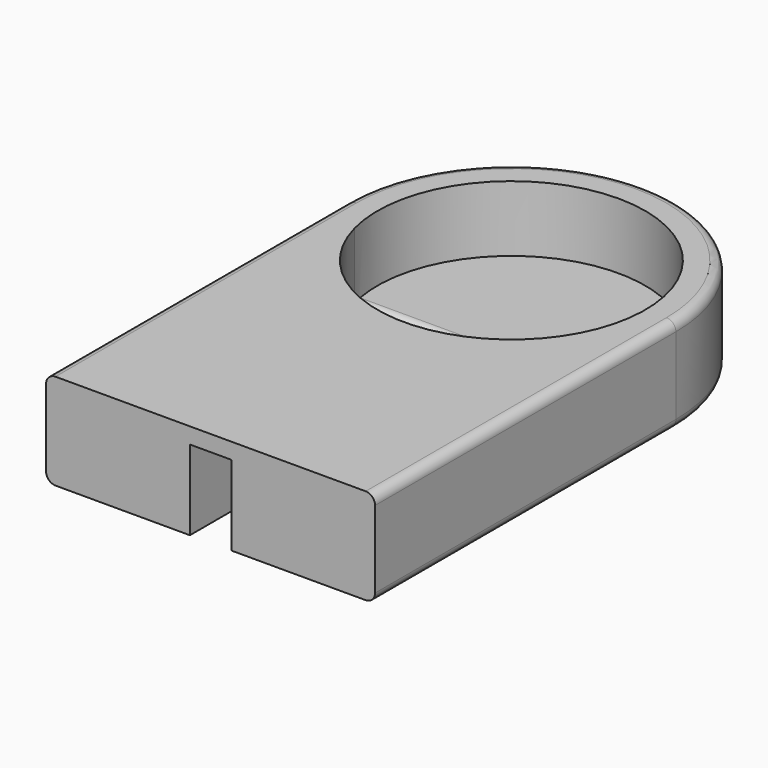
from build123d import *

# Parameters (mm, degrees)
F1_DEPTH     = 10.2
F2_R         = 14.25
F3_DEPTH     = 7
F4_W         = 4.4
F4_H         = 30
F5_DEPTH     = 8.5
F7_DEPTH     = 25
F9_T1_DEPTH  = 42.5
F9_T4_ANGLE  = 180
F9_T6_ANGLE  = 180
F9_T10_DEPTH = 32.5676095837
F9_S11_R     = 14.25
F9_T12_DEPTH = 18


# Not quite as in the source:
# - a fillet or chamfer that OpenCascade refuses, or shapes differently, is made with other operations: its cross-section is extruded or revolved along the edge and cut away or added


with BuildPart() as f1:
    # F0 (on Top) → F1 (new body)
    with BuildSketch(Plane.XY):
        with BuildLine():
            Line((-17.5, 20), (-17.5, -20))
            Line((-17.5, -20), (17.5, -20))
            Line((17.5, -20), (17.5, 20))
            ThreePointArc((17.5, 20), (0, 2.5), (-17.5, 20))
        make_face()
        with BuildLine():
            Line((17.5, 20), (-17.5, 20))
            ThreePointArc((-17.5, 20), (0, 2.5), (17.5, 20))
        make_face()
        with BuildLine():
            ThreePointArc((17.5, 20), (0, 37.5), (-17.5, 20))
            Line((-17.5, 20), (17.5, 20))
        make_face()
    extrude(amount=-F1_DEPTH)


with BuildPart() as f3:
    # F2 (on Top) → F3 (new body)
    with BuildSketch(Plane.XY):
        with Locations((0, 20)):
            Circle(F2_R)
    extrude(amount=-F3_DEPTH)


with BuildPart() as f5:
    # F4 (on face) → F5 (new body)
    with BuildSketch(Plane(origin=(0, 0, -10.2), x_dir=(1, 0, 0), z_dir=(0, 0, -1))):
        with Locations((0, 5)):
            Rectangle(F4_W, F4_H)
    extrude(amount=-F5_DEPTH)


with BuildPart() as f7:
    # F6 (on face) → F7 (new body)
    with BuildSketch(Plane(origin=(0, 0, -10.2), x_dir=(1, 0, 0), z_dir=(0, 0, -1))):
        with BuildLine():
            Line((-13.7838047919, -16.3848616264), (13.7838047919, -16.3848616264))
            ThreePointArc((13.7838047919, -16.3848616264), (0, -5.75), (-13.7838047919, -16.3848616264))
        make_face()
    extrude(amount=-F7_DEPTH)


with BuildPart() as f1_1:
    add(f1.part)

    # F8: cut F7, F5, F3
    add(f7.part, mode=Mode.SUBTRACT)
    add(f5.part, mode=Mode.SUBTRACT)
    add(f3.part, mode=Mode.SUBTRACT)

    # F9: fillet of radius 1 on 3 edges, made by hand

    # F9_s2 → F9_t1 (cut)
    with BuildSketch(Plane.XZ.offset(-20)):
        with BuildLine():
            ThreePointArc((16.5, -10.2), (17.2071067812, -9.9071067812), (17.5, -9.2))
            Line((17.5, -9.2), (17.5, -10.2))
            Line((17.5, -10.2), (16.5, -10.2))
        make_face()
        with BuildLine():
            ThreePointArc((-17.5, -9.2), (-17.2071067812, -9.9071067812), (-16.5, -10.2))
            Line((-16.5, -10.2), (-17.5, -10.2))
            Line((-17.5, -10.2), (-17.5, -9.2))
        make_face()
        with BuildLine():
            ThreePointArc((16.5, 0), (17.2071067812, -0.2928932188), (17.5, -1))
            Line((17.5, -1), (17.5, 0))
            Line((17.5, 0), (16.5, 0))
        make_face()
        with BuildLine():
            ThreePointArc((-17.5, -1), (-17.2071067812, -0.2928932188), (-16.5, 0))
            Line((-16.5, 0), (-17.5, 0))
            Line((-17.5, 0), (-17.5, -1))
        make_face()
    extrude(amount=F9_T1_DEPTH, mode=Mode.SUBTRACT)

    # F9_s3 → F9_t4 (revolve, cut)
    with BuildSketch(Plane.XZ.offset(-20)):
        with BuildLine():
            ThreePointArc((17.5, -1), (17.2071067812, -0.2928932188), (16.5, 0))
            Line((16.5, 0), (17.5, 0))
            Line((17.5, 0), (17.5, -1))
        make_face()
    revolve(axis=Axis((0, 20, 0), (0, 0, 1)), revolution_arc=F9_T4_ANGLE, mode=Mode.SUBTRACT)

    # F9_s5 → F9_t6 (revolve, cut)
    with BuildSketch(Plane.XZ.offset(-20)):
        with BuildLine():
            ThreePointArc((17.5, -9.2), (17.2071067812, -9.9071067812), (16.5, -10.2))
            Line((16.5, -10.2), (17.5, -10.2))
            Line((17.5, -10.2), (17.5, -9.2))
        make_face()
    revolve(axis=Axis((0, 20, -10.2), (0, 0, 1)), revolution_arc=F9_T6_ANGLE, mode=Mode.SUBTRACT)


with BuildPart() as f9_tool8:
    # F9_s9 → F9_t10 (new body)
    with BuildSketch(Plane.YZ.offset(-16.2838047919)):
        with BuildLine():
            ThreePointArc((16.3848616264, -8), (16.6777548452, -7.2928932188), (17.3848616264, -7))
            Line((17.3848616264, -7), (16.3848616264, -7))
            Line((16.3848616264, -7), (16.3848616264, -8))
        make_face()
    extrude(amount=F9_T10_DEPTH)

    # F9_s11 → F9_t12 (intersect, symmetric)
    with BuildSketch(Plane.XY.offset(-7.5)):
        with Locations((0, 20)):
            Circle(F9_S11_R)
    extrude(amount=F9_T12_DEPTH, both=True, mode=Mode.INTERSECT)


with BuildPart() as f1_2:
    add(f1_1.part)

    # F9_t7: cut F9_tool8
    add(f9_tool8.part, mode=Mode.SUBTRACT)


solid = f1_2.part
